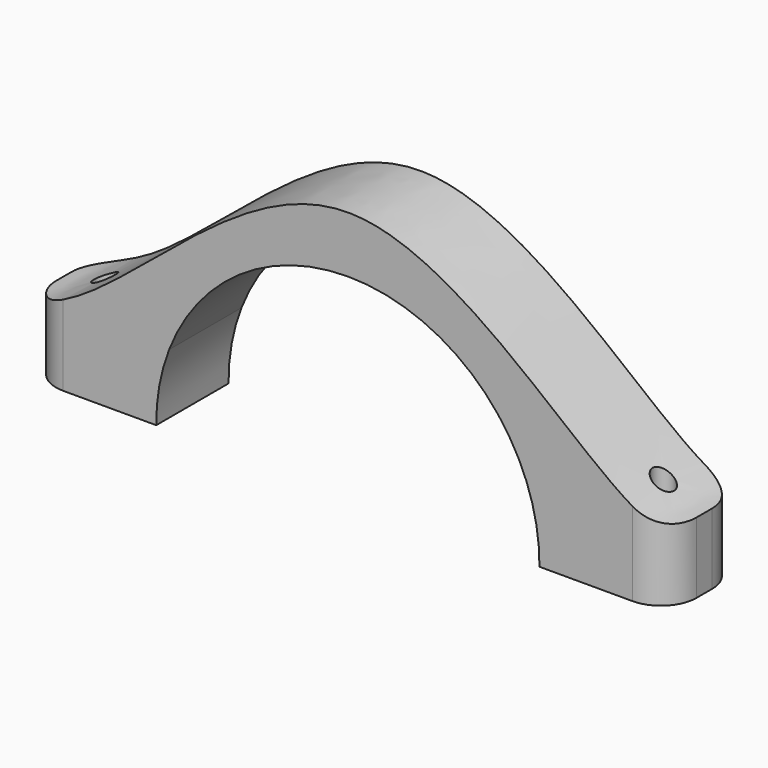
from build123d import *

# Parameters (mm, degrees)
F1_DEPTH = 12.7
F2_R     = 5
F3_R     = 1.5
F4_DEPTH = 15.1


# Not quite as in the source:
# - a feature names something its author has since deleted; it is built from what else it names


with BuildPart() as f1:
    # F0 (on Front) → F1 (new body)
    with BuildSketch(Plane.XZ):
        with BuildLine():
            Line((26.9239949913, -0.2326342749), (45, -0.2326342749))
            Line((45, -0.2326342749), (45, 9.7171152011))
            Line((45, 9.7171152011), (25.1104220827, 9.7171152011))
            ThreePointArc((25.1104220827, 9.7171152011), (26.4885733613, 4.828157649), (26.9239949913, -0.2326342749))
        make_face()
        with BuildLine():
            Line((25.1104220827, 9.7171152011), (45, 9.7171152011))
            add(Edge.make_bspline(
                [(-45, 9.7171152011), (-33.7651185691, 9.7171152011), (-1.2770984322, 59.9914556369), (36.3193154335, 9.7171152011), (45, 9.7171152011)],
                knots=[0, 0, 0, 0, 0.5, 1, 1, 1, 1], degree=3))
            Line((-45, 9.7171152011), (-25.1104220827, 9.7171152011))
            ThreePointArc((-25.1104220827, 9.7171152011), (0, 26.925), (25.1104220827, 9.7171152011))
        make_face()
        with BuildLine():
            Line((-25.1104220827, 9.7171152011), (-45, 9.7171152011))
            Line((-45, 9.7171152011), (-45, -0.2326342749))
            Line((-45, -0.2326342749), (-26.9239949913, -0.2326342749))
            ThreePointArc((-26.9239949913, -0.2326342749), (-26.4885733613, 4.828157649), (-25.1104220827, 9.7171152011))
        make_face()
    extrude(amount=F1_DEPTH)

    # F2
    f2_edges = [f1.edges().sort_by_distance(p)[0] for p in [
        (-45, -12.7, 4.74224),
        (-45, 0, 4.74224),
        (45, -12.7, 4.74224),
        (45, 0, 4.74224),
    ]]
    fillet(f2_edges, radius=F2_R)

    # F3 (on Top) → F4 (cut, symmetric)
    with BuildSketch(Plane.XY):
        with Locations((-39.25, -6.35)):
            Circle(F3_R)
        with Locations((39.25, -6.35)):
            Circle(F3_R)
    extrude(amount=F4_DEPTH, both=True, mode=Mode.SUBTRACT)


solid = f1.part
